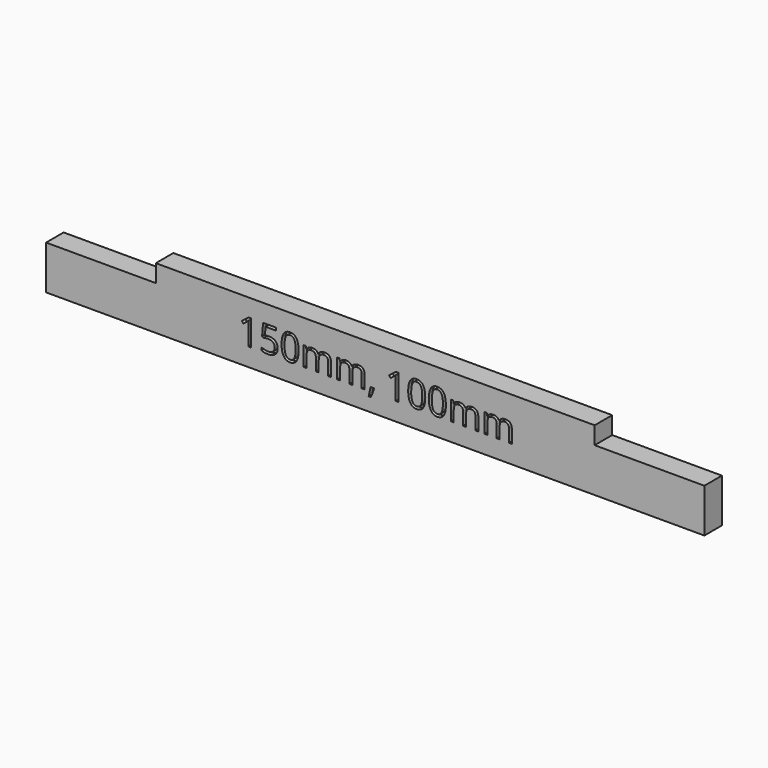
from build123d import *

# Parameters (mm, degrees)
F0_W         = 25
F0_H         = 5
F0_W_2       = 100
F1_DEPTH     = 10
F2_DEPTH     = 14
F3_TEXT_SIZE = 8.2238726059
F4_DEPTH     = 1
F5_TEXT_SIZE = 8.9524022769
F6_DEPTH     = 1


# Not quite as in the source:
# - Text() gives the source's letters only with a copy of the font that has no kerning and outlines rounded to 1/6400 em; it was checked with that copy


with BuildPart() as f1:
    # F0 (on Top) → F1 (new body)
    with BuildSketch(Plane.XY):
        with Locations((-62.5, -2.5)):
            Rectangle(F0_W, F0_H)
        with Locations((0, -2.5)):
            Rectangle(F0_W_2, F0_H)
        with Locations((62.5, -2.5)):
            Rectangle(F0_W, F0_H)
    extrude(amount=F1_DEPTH)

    # F0 (on Top) → F2 (join)
    with BuildSketch(Plane.XY):
        with Locations((0, -2.5)):
            Rectangle(F0_W_2, F0_H)
    extrude(amount=F2_DEPTH)

    # F3 (on face) → F4 (cut)
    with BuildSketch(Plane.XZ.offset(5)):
        with Locations((-31.1521468684, 4.1185212322)):
            Text('150mm, 100mm', F3_TEXT_SIZE, font='Open Sans', text_align=(TextAlign.LEFT, TextAlign.BOTTOM))
    extrude(amount=-F4_DEPTH, mode=Mode.SUBTRACT)

    # F5 (on face) → F6 (cut)
    with BuildSketch(Plane(origin=(0, 0, 0), x_dir=(-1, 0, 0), z_dir=(0, 1, 0))):
        with Locations((-40.9163720906, 3.5031142179)):
            Text('10mm , 14mm, 5mm', F5_TEXT_SIZE, font='Open Sans', text_align=(TextAlign.LEFT, TextAlign.BOTTOM))
    extrude(amount=-F6_DEPTH, mode=Mode.SUBTRACT)


solid = f1.part
